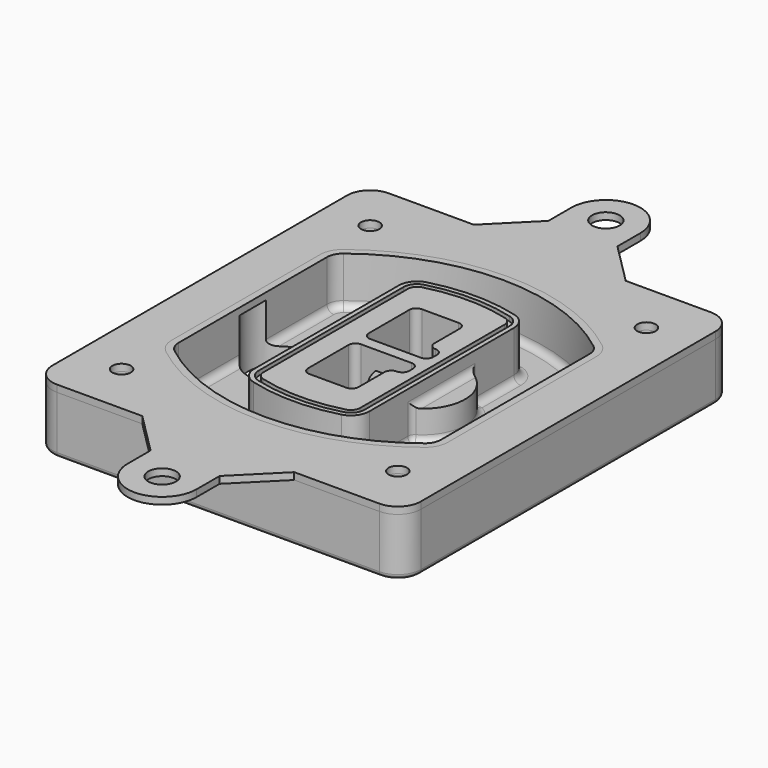
from build123d import *

# Parameters (mm, degrees)
F0_R      = 4
F1_DEPTH  = 25
F2_DEPTH  = 3
F3_DEPTH  = 18
F5_DEPTH  = 21
F6_DEPTH  = 2
F8_DEPTH  = 20
F9_DEPTH  = 16
F10_DEPTH = 25
F7_R      = 6
F7_R_2    = 4
F11_DEPTH = 6
F13_DEPTH = 9
F14_R     = 3
F15_R     = 2
F16_R     = 4
F16_R_2   = 6
F17_DEPTH = 3


with BuildPart() as f1:
    # F0 (on Top) → F1 (new body)
    with BuildSketch(Plane.XY):
        with BuildLine():
            ThreePointArc((-80, -80), (-77.0710678119, -87.0710678119), (-70, -90))
            Line((-70, -90), (70, -90))
            ThreePointArc((70, -90), (77.0710678119, -87.0710678119), (80, -80))
            Line((80, -80), (80, 80))
            ThreePointArc((80, 80), (77.0710678119, 87.0710678119), (70, 90))
            Line((70, 90), (-70, 90))
            ThreePointArc((-70, 90), (-77.0710678119, 87.0710678119), (-80, 80))
            Line((-80, 80), (-80, -80))
        make_face()
        with Locations((-60, -67.5)):
            Circle(F0_R, mode=Mode.SUBTRACT)
        with Locations((60, -67.5)):
            Circle(F0_R, mode=Mode.SUBTRACT)
        with Locations((-60, 67.5)):
            Circle(F0_R, mode=Mode.SUBTRACT)
        with BuildLine():
            ThreePointArc((-64, 40.2934422872), (-62.5820384798, 46.4328484224), (-58.6153846154, 51.3286200352))
            ThreePointArc((-58.6153846154, 51.3286200352), (0, 71.5), (58.6153846154, 51.3286200352))
            ThreePointArc((58.6153846154, 51.3286200352), (62.5820384798, 46.4328484224), (64, 40.2934422872))
            Line((64, 40.2934422872), (64, -40.2934422872))
            ThreePointArc((64, -40.2934422872), (62.5820384798, -46.4328484224), (58.6153846154, -51.3286200352))
            ThreePointArc((58.6153846154, -51.3286200352), (0, -71.5), (-58.6153846154, -51.3286200352))
            ThreePointArc((-58.6153846154, -51.3286200352), (-62.5820384798, -46.4328484224), (-64, -40.2934422872))
            Line((-64, -40.2934422872), (-64, 40.2934422872))
        make_face(mode=Mode.SUBTRACT)
        with Locations((60, 67.5)):
            Circle(F0_R, mode=Mode.SUBTRACT)
        with BuildLine():
            ThreePointArc((58.6153846154, 51.3286200352), (0, 71.5), (-58.6153846154, 51.3286200352))
            ThreePointArc((-58.6153846154, 51.3286200352), (-62.5820384798, 46.4328484224), (-64, 40.2934422872))
            Line((-64, 40.2934422872), (-64, -40.2934422872))
            ThreePointArc((-64, -40.2934422872), (-62.5820384798, -46.4328484224), (-58.6153846154, -51.3286200352))
            ThreePointArc((-58.6153846154, -51.3286200352), (0, -71.5), (58.6153846154, -51.3286200352))
            ThreePointArc((58.6153846154, -51.3286200352), (62.5820384798, -46.4328484224), (64, -40.2934422872))
            Line((64, -40.2934422872), (64, 40.2934422872))
            ThreePointArc((64, 40.2934422872), (62.5820384798, 46.4328484224), (58.6153846154, 51.3286200352))
        make_face()
        with BuildLine():
            Line((-60, -40.2934422872), (-60, 40.2934422872))
            ThreePointArc((-60, 40.2934422872), (-58.9871703427, 44.6787323838), (-56.1538461538, 48.1757121072))
            ThreePointArc((-56.1538461538, 48.1757121072), (0, 67.5), (56.1538461538, 48.1757121072))
            ThreePointArc((56.1538461538, 48.1757121072), (58.9871703427, 44.6787323838), (60, 40.2934422872))
            Line((60, 40.2934422872), (60, -40.2934422872))
            ThreePointArc((60, -40.2934422872), (58.9871703427, -44.6787323838), (56.1538461538, -48.1757121072))
            ThreePointArc((56.1538461538, -48.1757121072), (0, -67.5), (-56.1538461538, -48.1757121072))
            ThreePointArc((-56.1538461538, -48.1757121072), (-58.9871703427, -44.6787323838), (-60, -40.2934422872))
        make_face(mode=Mode.SUBTRACT)
        with BuildLine():
            ThreePointArc((-56.1538461538, 48.1757121072), (-58.9871703427, 44.6787323838), (-60, 40.2934422872))
            Line((-60, 40.2934422872), (-60, -40.2934422872))
            ThreePointArc((-60, -40.2934422872), (-58.9871703427, -44.6787323838), (-56.1538461538, -48.1757121072))
            ThreePointArc((-56.1538461538, -48.1757121072), (0, -67.5), (56.1538461538, -48.1757121072))
            ThreePointArc((56.1538461538, -48.1757121072), (58.9871703427, -44.6787323838), (60, -40.2934422872))
            Line((60, -40.2934422872), (60, 40.2934422872))
            ThreePointArc((60, 40.2934422872), (58.9871703427, 44.6787323838), (56.1538461538, 48.1757121072))
            ThreePointArc((56.1538461538, 48.1757121072), (0, 67.5), (-56.1538461538, 48.1757121072))
        make_face()
        with BuildLine():
            ThreePointArc((54.3076923077, 45.8110311612), (56.2910192399, 43.3631453548), (57, 40.2934422872))
            Line((57, 40.2934422872), (57, -40.2934422872))
            ThreePointArc((57, -40.2934422872), (56.2910192399, -43.3631453548), (54.3076923077, -45.8110311612))
            ThreePointArc((54.3076923077, -45.8110311612), (0, -64.5), (-54.3076923077, -45.8110311612))
            ThreePointArc((-54.3076923077, -45.8110311612), (-56.2910192399, -43.3631453548), (-57, -40.2934422872))
            Line((-57, -40.2934422872), (-57, 40.2934422872))
            ThreePointArc((-57, 40.2934422872), (-56.2910192399, 43.3631453548), (-54.3076923077, 45.8110311612))
            ThreePointArc((-54.3076923077, 45.8110311612), (0, 64.5), (54.3076923077, 45.8110311612))
        make_face(mode=Mode.SUBTRACT)
        with BuildLine():
            Line((57, -40.2934422872), (57, 40.2934422872))
            ThreePointArc((57, 40.2934422872), (56.2910192399, 43.3631453548), (54.3076923077, 45.8110311612))
            ThreePointArc((54.3076923077, 45.8110311612), (0, 64.5), (-54.3076923077, 45.8110311612))
            ThreePointArc((-54.3076923077, 45.8110311612), (-56.2910192399, 43.3631453548), (-57, 40.2934422872))
            Line((-57, 40.2934422872), (-57, -40.2934422872))
            ThreePointArc((-57, -40.2934422872), (-56.2910192399, -43.3631453548), (-54.3076923077, -45.8110311612))
            ThreePointArc((-54.3076923077, -45.8110311612), (0, -64.5), (54.3076923077, -45.8110311612))
            ThreePointArc((54.3076923077, -45.8110311612), (56.2910192399, -43.3631453548), (57, -40.2934422872))
        make_face()
    extrude(amount=-F1_DEPTH)

    # F0 (on Top) → F2 (join)
    with BuildSketch(Plane.XY):
        with BuildLine():
            ThreePointArc((-56.1538461538, 48.1757121072), (-58.9871703427, 44.6787323838), (-60, 40.2934422872))
            Line((-60, 40.2934422872), (-60, -40.2934422872))
            ThreePointArc((-60, -40.2934422872), (-58.9871703427, -44.6787323838), (-56.1538461538, -48.1757121072))
            ThreePointArc((-56.1538461538, -48.1757121072), (0, -67.5), (56.1538461538, -48.1757121072))
            ThreePointArc((56.1538461538, -48.1757121072), (58.9871703427, -44.6787323838), (60, -40.2934422872))
            Line((60, -40.2934422872), (60, 40.2934422872))
            ThreePointArc((60, 40.2934422872), (58.9871703427, 44.6787323838), (56.1538461538, 48.1757121072))
            ThreePointArc((56.1538461538, 48.1757121072), (0, 67.5), (-56.1538461538, 48.1757121072))
        make_face()
        with BuildLine():
            ThreePointArc((54.3076923077, 45.8110311612), (56.2910192399, 43.3631453548), (57, 40.2934422872))
            Line((57, 40.2934422872), (57, -40.2934422872))
            ThreePointArc((57, -40.2934422872), (56.2910192399, -43.3631453548), (54.3076923077, -45.8110311612))
            ThreePointArc((54.3076923077, -45.8110311612), (0, -64.5), (-54.3076923077, -45.8110311612))
            ThreePointArc((-54.3076923077, -45.8110311612), (-56.2910192399, -43.3631453548), (-57, -40.2934422872))
            Line((-57, -40.2934422872), (-57, 40.2934422872))
            ThreePointArc((-57, 40.2934422872), (-56.2910192399, 43.3631453548), (-54.3076923077, 45.8110311612))
            ThreePointArc((-54.3076923077, 45.8110311612), (0, 64.5), (54.3076923077, 45.8110311612))
        make_face(mode=Mode.SUBTRACT)
    extrude(amount=F2_DEPTH)

    # F0 (on Top) → F3 (cut)
    with BuildSketch(Plane.XY):
        with BuildLine():
            Line((57, -40.2934422872), (57, 40.2934422872))
            ThreePointArc((57, 40.2934422872), (56.2910192399, 43.3631453548), (54.3076923077, 45.8110311612))
            ThreePointArc((54.3076923077, 45.8110311612), (0, 64.5), (-54.3076923077, 45.8110311612))
            ThreePointArc((-54.3076923077, 45.8110311612), (-56.2910192399, 43.3631453548), (-57, 40.2934422872))
            Line((-57, 40.2934422872), (-57, -40.2934422872))
            ThreePointArc((-57, -40.2934422872), (-56.2910192399, -43.3631453548), (-54.3076923077, -45.8110311612))
            ThreePointArc((-54.3076923077, -45.8110311612), (0, -64.5), (54.3076923077, -45.8110311612))
            ThreePointArc((54.3076923077, -45.8110311612), (56.2910192399, -43.3631453548), (57, -40.2934422872))
        make_face()
    extrude(amount=-F3_DEPTH, mode=Mode.SUBTRACT)

    # F4 (on face) → F5 (join, through all)
    with BuildSketch(Plane.XY.offset(3)):
        with BuildLine():
            ThreePointArc((-25, -39.2465276821), (-23.3511545998, -44.1109737193), (-19.0842911877, -46.9702398883))
            ThreePointArc((-19.0842911877, -46.9702398883), (0, -49.5), (19.0842911877, -46.9702398883))
            ThreePointArc((19.0842911877, -46.9702398883), (23.3511545998, -44.1109737193), (25, -39.2465276821))
            Line((25, -39.2465276821), (25, 39.2465276821))
            ThreePointArc((25, 39.2465276821), (23.3511545998, 44.1109737193), (19.0842911877, 46.9702398883))
            ThreePointArc((19.0842911877, 46.9702398883), (0, 49.5), (-19.0842911877, 46.9702398883))
            ThreePointArc((-19.0842911877, 46.9702398883), (-23.3511545998, 44.1109737193), (-25, 39.2465276821))
            Line((-25, 39.2465276821), (-25, -39.2465276821))
        make_face()
        with BuildLine():
            ThreePointArc((18.5632183908, 45.0393118368), (21.7633659499, 42.89486221), (23, 39.2465276821))
            Line((23, 39.2465276821), (23, -39.2465276821))
            ThreePointArc((23, -39.2465276821), (21.7633659499, -42.89486221), (18.5632183908, -45.0393118368))
            ThreePointArc((18.5632183908, -45.0393118368), (0, -47.5), (-18.5632183908, -45.0393118368))
            ThreePointArc((-18.5632183908, -45.0393118368), (-21.7633659499, -42.89486221), (-23, -39.2465276821))
            Line((-23, -39.2465276821), (-23, 39.2465276821))
            ThreePointArc((-23, 39.2465276821), (-21.7633659499, 42.89486221), (-18.5632183908, 45.0393118368))
            ThreePointArc((-18.5632183908, 45.0393118368), (0, 47.5), (18.5632183908, 45.0393118368))
        make_face(mode=Mode.SUBTRACT)
        with BuildLine():
            Line((23, -39.2465276821), (23, 39.2465276821))
            ThreePointArc((23, 39.2465276821), (21.7633659499, 42.89486221), (18.5632183908, 45.0393118368))
            ThreePointArc((18.5632183908, 45.0393118368), (0, 47.5), (-18.5632183908, 45.0393118368))
            ThreePointArc((-18.5632183908, 45.0393118368), (-21.7633659499, 42.89486221), (-23, 39.2465276821))
            Line((-23, 39.2465276821), (-23, -39.2465276821))
            ThreePointArc((-23, -39.2465276821), (-21.7633659499, -42.89486221), (-18.5632183908, -45.0393118368))
            ThreePointArc((-18.5632183908, -45.0393118368), (0, -47.5), (18.5632183908, -45.0393118368))
            ThreePointArc((18.5632183908, -45.0393118368), (21.7633659499, -42.89486221), (23, -39.2465276821))
        make_face()
        with BuildLine():
            ThreePointArc((18.0421455939, 43.1083837852), (20.1755772999, 41.6787507007), (21, 39.2465276821))
            Line((21, 39.2465276821), (21, -39.2465276821))
            ThreePointArc((21, -39.2465276821), (20.1755772999, -41.6787507007), (18.0421455939, -43.1083837852))
            ThreePointArc((18.0421455939, -43.1083837852), (0, -45.5), (-18.0421455939, -43.1083837852))
            ThreePointArc((-18.0421455939, -43.1083837852), (-20.1755772999, -41.6787507007), (-21, -39.2465276821))
            Line((-21, -39.2465276821), (-21, 39.2465276821))
            ThreePointArc((-21, 39.2465276821), (-20.1755772999, 41.6787507007), (-18.0421455939, 43.1083837852))
            ThreePointArc((-18.0421455939, 43.1083837852), (0, 45.5), (18.0421455939, 43.1083837852))
        make_face(mode=Mode.SUBTRACT)
        with BuildLine():
            Line((21, -39.2465276821), (21, 39.2465276821))
            ThreePointArc((21, 39.2465276821), (20.1755772999, 41.6787507007), (18.0421455939, 43.1083837852))
            ThreePointArc((18.0421455939, 43.1083837852), (0, 45.5), (-18.0421455939, 43.1083837852))
            ThreePointArc((-18.0421455939, 43.1083837852), (-20.1755772999, 41.6787507007), (-21, 39.2465276821))
            Line((-21, 39.2465276821), (-21, -39.2465276821))
            ThreePointArc((-21, -39.2465276821), (-20.1755772999, -41.6787507007), (-18.0421455939, -43.1083837852))
            ThreePointArc((-18.0421455939, -43.1083837852), (0, -45.5), (18.0421455939, -43.1083837852))
            ThreePointArc((18.0421455939, -43.1083837852), (20.1755772999, -41.6787507007), (21, -39.2465276821))
        make_face()
        with BuildLine():
            Line((-8, -2.5), (14, -2.5))
            ThreePointArc((14, -2.5), (16.1213203436, -3.3786796564), (17, -5.5))
            Line((17, -5.5), (17, -7.5))
            ThreePointArc((17, -7.5), (16.1213203436, -9.6213203436), (14, -10.5))
            ThreePointArc((14, -10.5), (11.8786796564, -11.3786796564), (11, -13.5))
            Line((11, -13.5), (11, -27.5))
            ThreePointArc((11, -27.5), (10.1213203436, -29.6213203436), (8, -30.5))
            Line((8, -30.5), (-8, -30.5))
            ThreePointArc((-8, -30.5), (-10.1213203436, -29.6213203436), (-11, -27.5))
            Line((-11, -27.5), (-11, -5.5))
            ThreePointArc((-11, -5.5), (-10.1213203436, -3.3786796564), (-8, -2.5))
        make_face(mode=Mode.SUBTRACT)
        with BuildLine():
            ThreePointArc((-8, 2.5), (-10.1213203436, 3.3786796564), (-11, 5.5))
            Line((-11, 5.5), (-11, 27.5))
            ThreePointArc((-11, 27.5), (-10.1213203436, 29.6213203436), (-8, 30.5))
            Line((-8, 30.5), (8, 30.5))
            ThreePointArc((8, 30.5), (10.1213203436, 29.6213203436), (11, 27.5))
            Line((11, 27.5), (11, 13.5))
            ThreePointArc((11, 13.5), (11.8786796564, 11.3786796564), (14, 10.5))
            ThreePointArc((14, 10.5), (16.1213203436, 9.6213203436), (17, 7.5))
            Line((17, 7.5), (17, 5.5))
            ThreePointArc((17, 5.5), (16.1213203436, 3.3786796564), (14, 2.5))
            Line((14, 2.5), (-8, 2.5))
        make_face(mode=Mode.SUBTRACT)
    extrude(amount=-F5_DEPTH)

    # F4 (on face) → F6 (cut)
    with BuildSketch(Plane.XY.offset(3)):
        with BuildLine():
            Line((23, -39.2465276821), (23, 39.2465276821))
            ThreePointArc((23, 39.2465276821), (21.7633659499, 42.89486221), (18.5632183908, 45.0393118368))
            ThreePointArc((18.5632183908, 45.0393118368), (0, 47.5), (-18.5632183908, 45.0393118368))
            ThreePointArc((-18.5632183908, 45.0393118368), (-21.7633659499, 42.89486221), (-23, 39.2465276821))
            Line((-23, 39.2465276821), (-23, -39.2465276821))
            ThreePointArc((-23, -39.2465276821), (-21.7633659499, -42.89486221), (-18.5632183908, -45.0393118368))
            ThreePointArc((-18.5632183908, -45.0393118368), (0, -47.5), (18.5632183908, -45.0393118368))
            ThreePointArc((18.5632183908, -45.0393118368), (21.7633659499, -42.89486221), (23, -39.2465276821))
        make_face()
        with BuildLine():
            ThreePointArc((18.0421455939, 43.1083837852), (20.1755772999, 41.6787507007), (21, 39.2465276821))
            Line((21, 39.2465276821), (21, -39.2465276821))
            ThreePointArc((21, -39.2465276821), (20.1755772999, -41.6787507007), (18.0421455939, -43.1083837852))
            ThreePointArc((18.0421455939, -43.1083837852), (0, -45.5), (-18.0421455939, -43.1083837852))
            ThreePointArc((-18.0421455939, -43.1083837852), (-20.1755772999, -41.6787507007), (-21, -39.2465276821))
            Line((-21, -39.2465276821), (-21, 39.2465276821))
            ThreePointArc((-21, 39.2465276821), (-20.1755772999, 41.6787507007), (-18.0421455939, 43.1083837852))
            ThreePointArc((-18.0421455939, 43.1083837852), (0, 45.5), (18.0421455939, 43.1083837852))
        make_face(mode=Mode.SUBTRACT)
    extrude(amount=-F6_DEPTH, mode=Mode.SUBTRACT)

    # F7 (on face) → F8 (join)
    with BuildSketch(Plane(origin=(0, 0, -25), x_dir=(1, 0, 0), z_dir=(0, 0, -1))):
        with BuildLine():
            ThreePointArc((3.28842436, 0), (16.7567035675, 13.4682792075), (30.224982775, 0))
            Line((30.224982775, 0), (35.224982775, 0))
            ThreePointArc((35.224982775, 0), (16.7567035675, 18.4682792075), (-1.71157564, 0))
            Line((-1.71157564, 0), (3.28842436, 0))
        make_face()
        with BuildLine():
            Line((3.28842436, 0), (30.224982775, 0))
            ThreePointArc((30.224982775, 0), (16.7567035675, 13.4682792075), (3.28842436, 0))
        make_face()
        with BuildLine():
            ThreePointArc((3.28842436, 0), (16.7567035675, -13.4682792075), (30.224982775, 0))
            Line((30.224982775, 0), (3.28842436, 0))
        make_face()
        with BuildLine():
            Line((35.224982775, 0), (30.224982775, 0))
            ThreePointArc((30.224982775, 0), (16.7567035675, -13.4682792075), (3.28842436, 0))
            Line((3.28842436, 0), (-1.71157564, 0))
            ThreePointArc((-1.71157564, 0), (16.7567035675, -18.4682792075), (35.224982775, 0))
        make_face()
    extrude(amount=-F8_DEPTH)

    # F7 (on face) → F9 (cut)
    with BuildSketch(Plane(origin=(0, 0, -25), x_dir=(1, 0, 0), z_dir=(0, 0, -1))):
        with BuildLine():
            Line((3.28842436, 0), (30.224982775, 0))
            ThreePointArc((30.224982775, 0), (16.7567035675, 13.4682792075), (3.28842436, 0))
        make_face()
        with BuildLine():
            ThreePointArc((3.28842436, 0), (16.7567035675, -13.4682792075), (30.224982775, 0))
            Line((30.224982775, 0), (3.28842436, 0))
        make_face()
    extrude(amount=-F9_DEPTH, mode=Mode.SUBTRACT)

    # F7 (on face) → F10 (cut)
    with BuildSketch(Plane(origin=(0, 0, -25), x_dir=(1, 0, 0), z_dir=(0, 0, -1))):
        with BuildLine():
            Line((-59.0318229325, 0), (-32.0952645175, 0))
            ThreePointArc((-32.0952645175, 0), (-45.563543725, 13.4682792075), (-59.0318229325, 0))
        make_face()
        with BuildLine():
            ThreePointArc((-59.0318229325, 0), (-45.563543725, -13.4682792075), (-32.0952645175, 0))
            Line((-32.0952645175, 0), (-59.0318229325, 0))
        make_face()
    extrude(amount=-F10_DEPTH, mode=Mode.SUBTRACT)

    # F7 (on face) → F11 (cut)
    with BuildSketch(Plane(origin=(0, 0, -25), x_dir=(1, 0, 0), z_dir=(0, 0, -1))):
        with Locations((60, -67.5)):
            Circle(F7_R)
        with Locations((60, -67.5)):
            Circle(F7_R_2, mode=Mode.SUBTRACT)
        with Locations((-60, -67.5)):
            Circle(F7_R)
        with Locations((-60, -67.5)):
            Circle(F7_R_2, mode=Mode.SUBTRACT)
        with Locations((-60, 67.5)):
            Circle(F7_R)
        with Locations((-60, 67.5)):
            Circle(F7_R_2, mode=Mode.SUBTRACT)
        with Locations((60, 67.5)):
            Circle(F7_R)
        with Locations((60, 67.5)):
            Circle(F7_R_2, mode=Mode.SUBTRACT)
    extrude(amount=-F11_DEPTH, mode=Mode.SUBTRACT)

    # F12 (on face) → F13 (cut, through all)
    with BuildSketch(Plane(origin=(0, 0, -9), x_dir=(1, 0, 0), z_dir=(0, 0, -1))):
        with BuildLine():
            Line((11, 13.5), (11, 17.5481537753))
            ThreePointArc((11, 17.5481537753), (2.5696536419, 11.8239143813), (-1.5415842455, 2.5))
            Line((-1.5415842455, 2.5), (3.5224848595, 2.5))
            ThreePointArc((3.5224848595, 2.5), (6.1857188154, 8.3455872281), (11.2536447004, 12.2927168648))
            ThreePointArc((11.2536447004, 12.2927168648), (11.0640958889, 12.8831798879), (11, 13.5))
        make_face()
        with BuildLine():
            ThreePointArc((11.2536447004, -12.2927168648), (6.1857188154, -8.3455872281), (3.5224848595, -2.5))
            Line((3.5224848595, -2.5), (-1.5415842455, -2.5))
            ThreePointArc((-1.5415842455, -2.5), (2.5696536419, -11.8239143813), (11, -17.5481537753))
            Line((11, -17.5481537753), (11, -13.5))
            ThreePointArc((11, -13.5), (11.0640958889, -12.8831798879), (11.2536447004, -12.2927168648))
        make_face()
        with BuildLine():
            ThreePointArc((11.2536447004, 12.2927168648), (6.1857188154, 8.3455872281), (3.5224848595, 2.5))
            Line((3.5224848595, 2.5), (14, 2.5))
            ThreePointArc((14, 2.5), (16.1213203436, 3.3786796564), (17, 5.5))
            Line((17, 5.5), (17, 7.5))
            ThreePointArc((17, 7.5), (16.1213203436, 9.6213203436), (14, 10.5))
            ThreePointArc((14, 10.5), (12.3601599782, 10.9878446101), (11.2536447004, 12.2927168648))
        make_face()
        with BuildLine():
            Line((14, -2.5), (3.5224848595, -2.5))
            ThreePointArc((3.5224848595, -2.5), (6.1857188154, -8.3455872281), (11.2536447004, -12.2927168648))
            ThreePointArc((11.2536447004, -12.2927168648), (12.3601599782, -10.9878446101), (14, -10.5))
            ThreePointArc((14, -10.5), (16.1213203436, -9.6213203436), (17, -7.5))
            Line((17, -7.5), (17, -5.5))
            ThreePointArc((17, -5.5), (16.1213203436, -3.3786796564), (14, -2.5))
        make_face()
    extrude(amount=F13_DEPTH, mode=Mode.SUBTRACT)

    # F14
    f14_edges = [f1.edges().sort_by_distance(p)[0] for p in [
        (-57, -23.703476, -18),
        (-57, 23.703476, -18),
        (25, 0, -5),
        (25, 16.526506, -11.5),
        (25, -16.526506, -11.5),
        (25, -27.886517, -18),
        (35.224983, 0, -18),
    ]]
    fillet(f14_edges, radius=F14_R)

    # F15
    f15_edges = [f1.edges().sort_by_distance(p)[0] for p in [
        (0, -90, -25),
    ]]
    fillet(f15_edges, radius=F15_R)


with BuildPart() as f17:
    # F16 (on face) → F17 (new body, through all)
    with BuildSketch(Plane.XY):
        with BuildLine():
            Line((-80, 80), (-80, -80))
            ThreePointArc((-80, -80), (-77.0710678119, -87.0710678119), (-70, -90))
            Line((-70, -90), (-36.5033634007, -90))
            Line((-36.5033634007, -90), (-32.9932081352, -90))
            Line((-32.9932081352, -90), (33, -90))
            Line((33, -90), (70, -90))
            ThreePointArc((70, -90), (77.0710678119, -87.0710678119), (80, -80))
            Line((80, -80), (80, 80))
            ThreePointArc((80, 80), (77.0710678119, 87.0710678119), (70, 90))
            Line((70, 90), (33, 90))
            Line((33, 90), (-32.9932081352, 90))
            Line((-32.9932081352, 90), (-36.5033634007, 90))
            Line((-36.5033634007, 90), (-70, 90))
            ThreePointArc((-70, 90), (-77.0710678119, 87.0710678119), (-80, 80))
        make_face()
        with Locations((-60, -67.5)):
            Circle(F16_R, mode=Mode.SUBTRACT)
        with Locations((60, -67.5)):
            Circle(F16_R, mode=Mode.SUBTRACT)
        with Locations((-60, 67.5)):
            Circle(F16_R, mode=Mode.SUBTRACT)
        with BuildLine():
            ThreePointArc((56.1538461538, -48.1757121072), (0, -67.5), (-56.1538461538, -48.1757121072))
            ThreePointArc((-56.1538461538, -48.1757121072), (-58.9871703427, -44.6787323838), (-60, -40.2934422872))
            Line((-60, -40.2934422872), (-60, 40.2934422872))
            ThreePointArc((-60, 40.2934422872), (-58.9871703427, 44.6787323838), (-56.1538461538, 48.1757121072))
            ThreePointArc((-56.1538461538, 48.1757121072), (0, 67.5), (56.1538461538, 48.1757121072))
            ThreePointArc((56.1538461538, 48.1757121072), (58.9871703427, 44.6787323838), (60, 40.2934422872))
            Line((60, 40.2934422872), (60, -40.2934422872))
            ThreePointArc((60, -40.2934422872), (58.9871703427, -44.6787323838), (56.1538461538, -48.1757121072))
        make_face(mode=Mode.SUBTRACT)
        with Locations((60, 67.5)):
            Circle(F16_R, mode=Mode.SUBTRACT)
        with BuildLine():
            Line((33, -90), (-32.9932081352, -90))
            Line((-32.9932081352, -90), (-14.9932081352, -108))
            Line((-14.9932081352, -108), (-14.9932081352, -120))
            ThreePointArc((-14.9932081352, -120), (-0.2256966684, -135.4496441749), (15, -120.4513422372))
            Line((15, -120.4513422372), (15, -108))
            Line((15, -108), (33, -90))
        make_face()
        with Locations((0, -120.4513422372)):
            Circle(F16_R_2, mode=Mode.SUBTRACT)
        with BuildLine():
            Line((-14.9932081352, 108), (-32.9932081352, 90))
            Line((-32.9932081352, 90), (33, 90))
            Line((33, 90), (15, 108))
            Line((15, 108), (15, 120.4513422372))
            ThreePointArc((15, 120.4513422372), (-0.2256966684, 135.4496441749), (-14.9932081352, 120))
            Line((-14.9932081352, 120), (-14.9932081352, 108))
        make_face()
        with Locations((0, 120.4513422372)):
            Circle(F16_R_2, mode=Mode.SUBTRACT)
    extrude(amount=F17_DEPTH)


solid = Compound([f1.part, f17.part])
